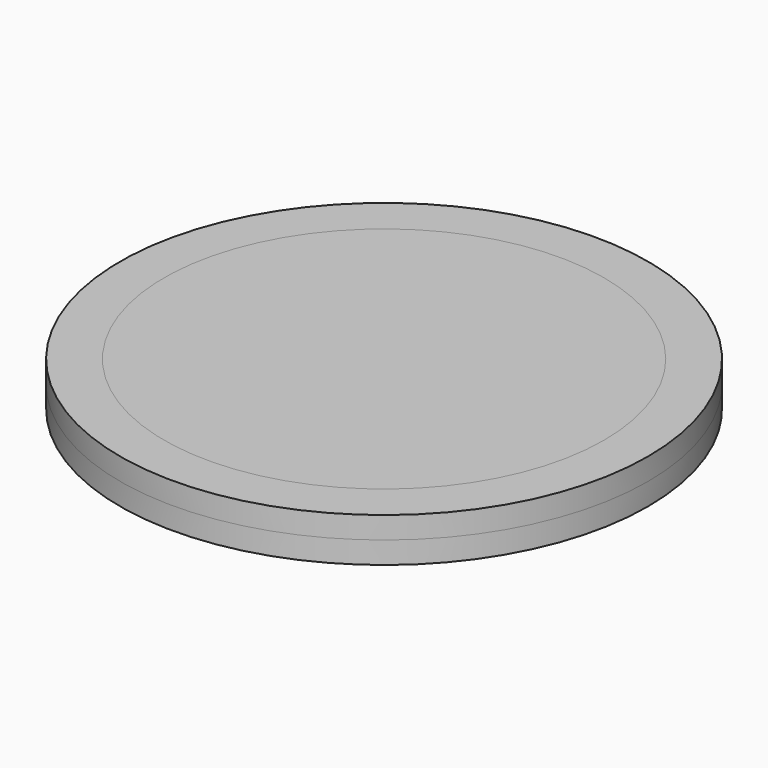
from build123d import *

# Parameters (mm, degrees)
F0_R      = 38.1
F1_DEPTH  = 3.175
F2_DEPTH  = 3.175
F3_R      = 38.1
F3_R_2    = 31.75
F4_DEPTH  = 3.175
F5_R      = 38.1
F5_R_2    = 31.75
F6_DEPTH  = 3.175
F8_DEPTH  = 3.175
F10_DEPTH = 3.175


with BuildPart() as f1:
    # F0 (on Top) → F1 (new body)
    with BuildSketch(Plane.XY):
        Circle(F0_R)
    extrude(amount=F1_DEPTH)

    # F3 (on face) → F4 (cut, through all)
    with BuildSketch(Plane.XY.offset(3.175)):
        Circle(F3_R)
        Circle(F3_R_2, mode=Mode.SUBTRACT)
    extrude(amount=-F4_DEPTH, mode=Mode.SUBTRACT)

    # F9 (on face) → F10 (join, through all)
    with BuildSketch(Plane.XY):
        Polygon((-13.4703841816, -22.4506403027), (0, -8.9802561211), (13.4703841816, -22.4506403027), (22.4506403027, -13.4703841816), (8.9802561211, 0), (22.4506403027, 13.4703841816), (13.4703841816, 22.4506403027), (0, 8.9802561211), (-13.4703841816, 22.4506403027), (-22.4506403027, 13.4703841816), (-8.9802561211, 0), (-22.4506403027, -13.4703841816), align=None)
    extrude(amount=-F10_DEPTH)


with BuildPart() as f2:
    # F0 (on Top) → F2 (new body)
    with BuildSketch(Plane.XY):
        Circle(F0_R)
    extrude(amount=-F2_DEPTH)

    # F5 (on face) → F6 (join, through all)
    with BuildSketch(Plane.XY):
        Circle(F5_R)
        Circle(F5_R_2, mode=Mode.SUBTRACT)
    extrude(amount=F6_DEPTH)

    # F7 (on face) → F8 (cut, through all)
    with BuildSketch(Plane(origin=(0, 0, -3.175), x_dir=(1, 0, 0), z_dir=(0, 0, -1))):
        Polygon((13.4703841816, 22.4506403027), (0, 8.9802561211), (-13.4703841816, 22.4506403027), (-22.4506403027, 13.4703841816), (-8.9802561211, 0), (-22.4506403027, -13.4703841816), (-13.4703841816, -22.4506403027), (0, -8.9802561211), (13.4703841816, -22.4506403027), (22.4506403027, -13.4703841816), (8.9802561211, 0), (22.4506403027, 13.4703841816), align=None)
    extrude(amount=-F8_DEPTH, mode=Mode.SUBTRACT)


solid = Compound([f1.part, f2.part])
